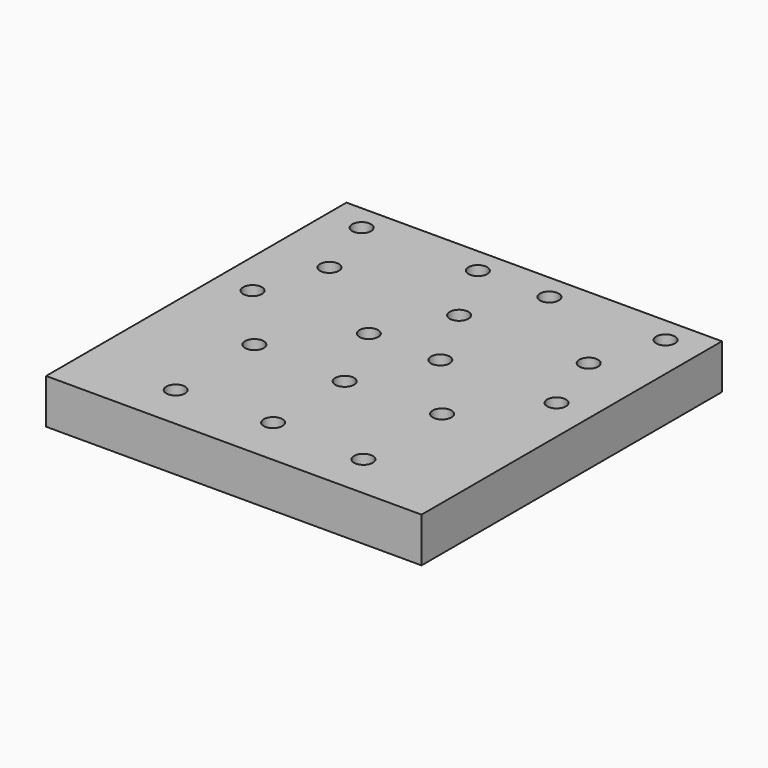
from build123d import *

# Parameters (mm, degrees)
F0_W           = 84
F0_H           = 84
F1_DEPTH       = 10
F3_D           = 4.2
F5_D           = 4.2
F5_CBORE_D     = 9.75
F5_CBORE_DEPTH = 5


# Not quite as in the source:
# - a feature names something its author has since deleted; it is built from what else it names


with BuildPart() as f1:
    # F0 (on Top) → F1 (new body)
    with BuildSketch(Plane.XY):
        Rectangle(F0_W, F0_H)
    extrude(amount=F1_DEPTH)

    # F3 (through all)
    with Locations(Plane.XY.offset(10)):
        with Locations((-34, 36.25), (-8, 36.25), (8, 36.25), (34, 36.25), (34, 5.75), (8, 5.75), (-8, 5.75), (-34, 5.75), (0, -11), (0, -31)):
            Hole(F3_D / 2)

    # F5 (through all)
    with Locations(Plane(origin=(0, 0, 0), x_dir=(1, 0, 0), z_dir=(0, 0, -1))):
        with Locations((29, -21), (0, -21), (-29, -21), (21, 10), (21, 32), (-21, 32), (-21, 10)):
            CounterBoreHole(F5_D / 2, F5_CBORE_D / 2, F5_CBORE_DEPTH)


solid = f1.part
